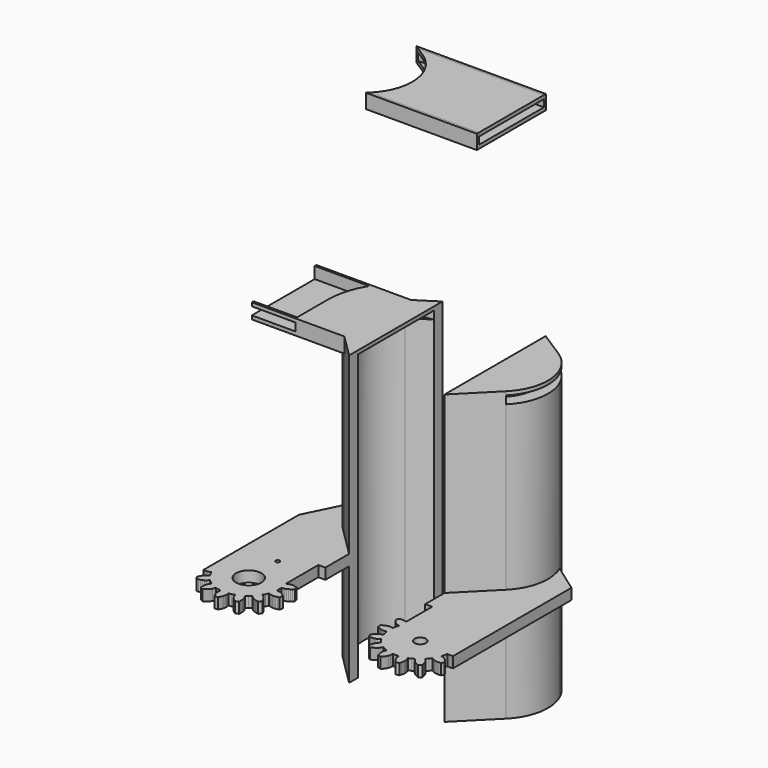
from build123d import *

# Parameters (mm, degrees)
F1_DEPTH  = 1.5
F0_R      = 1.6
F2_DEPTH  = 50
F3_DEPTH  = 30
F4_DEPTH  = 49
F5_DEPTH  = 46.8
F6_DEPTH  = 46.8
F7_DEPTH  = 45.8
F8_DEPTH  = 49
F9_DEPTH  = 45.8
F10_DEPTH = 1.5
F12_DEPTH = 4
F13_DEPTH = 3
F14_DEPTH = 1


# Not quite as in the source:
# - ends of sketch curves that miss each other by under 0.0002 mm in the source are joined
# - a feature names something its author has since deleted; it is built from what else it names


with BuildPart() as f1:
    # F0 (on Top) → F1 (new body, symmetric)
    with BuildSketch(Plane.XY):
        Polygon((-12.6828804, -37.9996929195), (-11.8884367355, -38.2222305677), (-11.8880267366, -38.2224279172), (-11.075543, -38.3664943195), (-11.1792258, -39.1773131195), (-11.1500412, -39.5862277195), (-11.049381, -40.0020257195), (-10.8967016, -40.4206431195), (-10.6978958, -40.8390065195), (-10.4565196, -41.2543727195), (-9.5434404, -41.2543727195), (-9.302115, -40.8390065195), (-9.1033092, -40.4206431195), (-8.950579, -40.0020257195), (-8.8499188, -39.5862277195), (-8.820785, -39.1773131195), (-8.9244678, -38.3664943195), (-8.1119840634, -38.2224279172), (-8.1115408, -38.2223493195), (-7.3171558, -37.9996929195), (-7.0589394, -38.7751549195), (-6.8550028, -39.1308311195), (-6.5838324, -39.4619201195), (-6.2647068, -39.7727145195), (-5.9041792, -40.0633667195), (-5.5066184, -40.3329369195), (-4.6838108, -39.9365445195), (-4.646549, -39.4578053195), (-4.6491144, -38.9947125195), (-4.693031, -38.5513555195), (-4.7828454, -38.1327635195), (-4.9339246, -37.7516365195), (-5.3789072, -37.0664715195), (-4.7096916266, -36.5840362135), (-4.709287, -36.5837445195), (-4.0899842, -36.0385589195), (-3.5209988, -36.6249941195), (-3.1831534, -36.8570993195), (-2.7948636, -37.0377695195), (-2.3725632, -37.1791713195), (-1.9218148, -37.2846829195), (-1.4464538, -37.3550663195), (-0.8770112, -36.6409453195), (-1.0512806, -36.1933973195), (-1.2544552, -35.7773199195), (-1.4865096, -35.3969041195), (-1.7489424, -35.0588555195), (-2.0504658, -34.7809287195), (-2.7488388, -34.3565455195), (-2.3551745142, -33.6315615111), (-2.3549356, -33.6311215195), (-2.0336002, -32.8714075195), (-1.2662154, -33.1527887195), (-0.86106, -33.2152727195), (-0.4331716, -33.2096847195), (0.0087884, -33.1539317195), (0.4607052, -33.0533223195), (0.9195562, -32.9104727195), (1.1227562, -32.0200757195), (0.7714742, -31.6924411195), (0.4079494, -31.4057259195), (0.033782, -31.1636639195), (-0.3494024, -30.9728083195), (-0.741426, -30.8533775195), (-1.5548356, -30.7739771195), (-1.5148031909, -29.9499745831), (-1.5147798, -29.9494931195), (-1.5548356, -29.1254663195), (-0.741426, -29.0460913195), (-0.3494024, -28.9266605195), (0.033782, -28.7358049195), (0.4079494, -28.4937683195), (0.7714742, -28.2070531195), (1.1227562, -27.8793931195), (0.9195562, -26.9889961195), (0.4607052, -26.8461465195), (0.0087884, -26.7455371195), (-0.4331716, -26.6898095195), (-0.86106, -26.6842215195), (-1.2662154, -26.7467055195), (-1.999996, -27.0157423195), (-1.999996, -15.8072914928), (-0.05, -15.8072914928), (-0.05, -8.999886363), (-7.8088611939, -1.2753778), (-20.002250767, -1.2753778), (-20.0087992, -33.1539317195), (-19.5667884, -33.2096847195), (-19.1389, -33.2152727195), (-18.7337954, -33.1527887195), (-17.9664106, -32.8714075195), (-17.6450069939, -33.6311141557), (-17.6448212, -33.6315533195), (-17.251172, -34.3565455195), (-17.9495196, -34.7809287195), (-18.2510684, -35.0588555195), (-18.5134504, -35.3969041195), (-18.745581, -35.7773199195), (-18.9487302, -36.1933973195), (-19.1229996, -36.6409453195), (-18.5535062, -37.3550663195), (-18.078196, -37.2846829195), (-17.6274476, -37.1791713195), (-17.2051218, -37.0377695195), (-16.8168066, -36.8570993195), (-16.479012, -36.6249941195), (-15.9100012, -36.0385589195), (-15.2906723648, -36.583686083), (-15.2903174, -36.5839985195), (-14.6211036, -37.0664715195), (-15.0660862, -37.7516365195), (-15.2171654, -38.1327635195), (-15.306929, -38.5513555195), (-15.3509218, -38.9947125195), (-15.3534618, -39.4578053195), (-15.3162, -39.9365445195), (-14.493367, -40.3329369195), (-14.0958062, -40.0633667195), (-13.735304, -39.7727145195), (-13.4161784, -39.4619201195), (-13.1449572, -39.1308311195), (-12.9410968, -38.7751549195), align=None)
        with BuildLine():
            ThreePointArc((-9.99998, -26.4247471195), (-7.5074285963, -27.4571957159), (-6.47498, -29.9497471195))
            ThreePointArc((-6.47498, -29.9497471195), (-12.4925314037, -32.4422985232), (-9.99998, -26.4247471195))
        make_face(mode=Mode.SUBTRACT)
        with BuildLine():
            ThreePointArc((-9.4549722, -19.9497471195), (-9.6146012888, -20.3351258307), (-9.99998, -20.4947549195))
            ThreePointArc((-9.99998, -20.4947549195), (-10.3853587112, -19.5643684084), (-9.4549722, -19.9497471195))
        make_face(mode=Mode.SUBTRACT)
        Polygon((-6.3914999282, -1.2753778), (-7.8088611939, -1.2753778), (-0.05, -8.999886363), (-0.05, -7.5888005143), align=None)
        Polygon((-8.4115295291, -0.6753778), (-7.8088611939, -1.2753778), (-6.3914999282, -1.2753778), (-6.9941682635, -0.6753778), align=None)
        with BuildLine():
            Line((-17.0059758203, 6.0612871152), (-17.0059758203, -0.6753778))
            Line((-17.0059758203, -0.6753778), (-8.4115295291, -0.6753778))
            Line((-8.4115295291, -0.6753778), (-6.9941682635, -0.6753778))
            Line((-6.9941682635, -0.6753778), (-8.8192027426, 1.1415762748))
            ThreePointArc((-8.8192027426, 1.1415762748), (-12.4595999549, 8.9958202972), (-10.1240431199, 17.331695494))
            Line((-10.1240431199, 17.331695494), (-12.1022985118, 15.9820039061))
            Line((-12.1022985118, 15.9820039061), (-17.0059758203, 6.0612871152))
        make_face()
        Polygon((-20.0019887813, 0), (-20.0021275162, -0.6753778), (-17.0059758203, -0.6753778), (-17.0059758203, 6.0612871152), align=None)
        Polygon((-20.0021275162, -0.6753778), (-20.002250767, -1.2753778), (-7.8088611939, -1.2753778), (-8.4115295291, -0.6753778), (-17.0059758203, -0.6753778), align=None)
    extrude(amount=F1_DEPTH, both=True)

    # F0 (on Top) → F2 (join)
    with BuildSketch(Plane.XY):
        with BuildLine():
            Line((-8.8192027426, 1.1415762748), (-6.9941682635, -0.6753778))
            Line((-6.9941682635, -0.6753778), (-0.05, -4.5405198881))
            Line((-0.05, -4.5405198881), (-7.28327834, 3.1477115777))
            ThreePointArc((-7.28327834, 3.1477115777), (-9.9219987158, 11.2465718924), (-5.3618740808, 18.4409896542))
            Line((-5.3618740808, 18.4409896542), (-0.05, 21.8151911543))
            Line((-0.05, 21.8151911543), (-6.7420944452, 20.5258809799))
            ThreePointArc((-6.7420944452, 20.5258809799), (-8.5829688524, 19.0874998536), (-10.1240431199, 17.331695494))
            ThreePointArc((-10.1240431199, 17.331695494), (-12.4595999549, 8.9958202972), (-8.8192027426, 1.1415762748))
        make_face()
        Polygon((-5.8053634872, 21.1258809799), (-6.7420944452, 20.5258809799), (-0.05, 21.8151911543), (-0.05, 22.999886363), (-0.05, 24.8123376548), align=None)
        Polygon((-6.9941682635, -0.6753778), (-6.3914999282, -1.2753778), (-0.05, -7.5888005143), (-0.05, -5.999886363), (-0.05, -4.5405198881), align=None)
        with BuildLine():
            Line((-7.28327834, 3.1477115777), (-0.05, -4.5405198881))
            Line((-0.05, -4.5405198881), (-0.05, 21.8151911543))
            Line((-0.05, 21.8151911543), (-5.3618740808, 18.4409896542))
            ThreePointArc((-5.3618740808, 18.4409896542), (-9.9219987158, 11.2465718924), (-7.28327834, 3.1477115777))
        make_face()
        with BuildLine():
            Line((-17.0059758203, 20.5258809799), (-17.0059758203, 6.0612871152))
            Line((-17.0059758203, 6.0612871152), (-12.1022985118, 15.9820039061))
            Line((-12.1022985118, 15.9820039061), (-10.1240431199, 17.331695494))
            ThreePointArc((-10.1240431199, 17.331695494), (-8.5829688524, 19.0874998536), (-6.7420944452, 20.5258809799))
            Line((-6.7420944452, 20.5258809799), (-17.0059758203, 20.5258809799))
        make_face()
        with BuildLine():
            Line((-19.9999346, 10), (-20.0019887813, 0))
            Line((-20.0019887813, 0), (-17.0059758203, 6.0612871152))
            Line((-17.0059758203, 6.0612871152), (-17.0059758203, 20.5258809799))
            ThreePointArc((-17.0059758203, 20.5258809799), (-19.2368888885, 15.4716989952), (-19.9999346, 10))
        make_face()
        Polygon((-20.0019887813, 0), (-20.0021275162, -0.6753778), (-17.0059758203, -0.6753778), (-17.0059758203, 6.0612871152), align=None)
        with BuildLine():
            Line((-17.0059758203, 6.0612871152), (-17.0059758203, -0.6753778))
            Line((-17.0059758203, -0.6753778), (-8.4115295291, -0.6753778))
            Line((-8.4115295291, -0.6753778), (-6.9941682635, -0.6753778))
            Line((-6.9941682635, -0.6753778), (-8.8192027426, 1.1415762748))
            ThreePointArc((-8.8192027426, 1.1415762748), (-12.4595999549, 8.9958202972), (-10.1240431199, 17.331695494))
            Line((-10.1240431199, 17.331695494), (-12.1022985118, 15.9820039061))
            Line((-12.1022985118, 15.9820039061), (-17.0059758203, 6.0612871152))
        make_face()
        with BuildLine():
            ThreePointArc((-16.6196316573, 21.1258809799), (-16.8154800574, 20.82760428), (-17.0059758203, 20.5258809799))
            Line((-17.0059758203, 20.5258809799), (-6.7420944452, 20.5258809799))
            Line((-6.7420944452, 20.5258809799), (-5.8053634872, 21.1258809799))
            Line((-5.8053634872, 21.1258809799), (-16.6196316573, 21.1258809799))
        make_face()
        Polygon((-8.4115295291, -0.6753778), (-7.8088611939, -1.2753778), (-6.3914999282, -1.2753778), (-6.9941682635, -0.6753778), align=None)
        Polygon((-20.0021275162, -0.6753778), (-20.002250767, -1.2753778), (-7.8088611939, -1.2753778), (-8.4115295291, -0.6753778), (-17.0059758203, -0.6753778), align=None)
        with BuildLine():
            Line((-27.5000003164, 20.5258809799), (-17.0059758203, 20.5258809799))
            ThreePointArc((-17.0059758203, 20.5258809799), (-16.8154800574, 20.82760428), (-16.6196316573, 21.1258809799))
            Line((-16.6196316573, 21.1258809799), (-27.5000003164, 21.1258809799))
            Line((-27.5000003164, 21.1258809799), (-32.0804677904, 21.1258809799))
            Line((-32.0804677904, 21.1258809799), (-32.0804677904, 20.5258809799))
            Line((-32.0804677904, 20.5258809799), (-27.5000003164, 20.5258809799))
        make_face()
        Polygon((-27.5000003164, -1.2753778), (-20.002250767, -1.2753778), (-20.0021275162, -0.6753778), (-27.5000003164, -0.6753778), (-32.0804677904, -0.6753778), (-32.0804677904, -1.2753778), align=None)
    extrude(amount=F2_DEPTH)

    # F0 (on Top) → F3 (join)
    with BuildSketch(Plane.XY):
        with BuildLine():
            Line((-8.8192027426, 1.1415762748), (-6.9941682635, -0.6753778))
            Line((-6.9941682635, -0.6753778), (-0.05, -4.5405198881))
            Line((-0.05, -4.5405198881), (-7.28327834, 3.1477115777))
            ThreePointArc((-7.28327834, 3.1477115777), (-9.9219987158, 11.2465718924), (-5.3618740808, 18.4409896542))
            Line((-5.3618740808, 18.4409896542), (-0.05, 21.8151911543))
            Line((-0.05, 21.8151911543), (-6.7420944452, 20.5258809799))
            ThreePointArc((-6.7420944452, 20.5258809799), (-8.5829688524, 19.0874998536), (-10.1240431199, 17.331695494))
            ThreePointArc((-10.1240431199, 17.331695494), (-12.4595999549, 8.9958202972), (-8.8192027426, 1.1415762748))
        make_face()
        Polygon((-6.9941682635, -0.6753778), (-6.3914999282, -1.2753778), (-0.05, -7.5888005143), (-0.05, -5.999886363), (-0.05, -4.5405198881), align=None)
        Polygon((-5.8053634872, 21.1258809799), (-6.7420944452, 20.5258809799), (-0.05, 21.8151911543), (-0.05, 22.999886363), (-0.05, 24.8123376548), align=None)
    extrude(amount=-F3_DEPTH)


with BuildPart() as f1b:
    # F0 (on Top) → F1, piece 2 (new body, symmetric)
    with BuildSketch(Plane.XY):
        with BuildLine():
            Line((45.5568809356, -32.5242657195), (45.7794119864, -31.729845607))
            Line((45.7794119864, -31.729845607), (45.7796203111, -31.7294128346))
            Line((45.7796203111, -31.7294128346), (45.9237077356, -30.9169283195))
            Line((45.9237077356, -30.9169283195), (46.7345011356, -31.0206111195))
            Line((46.7345011356, -31.0206111195), (47.1434157356, -30.9914519195))
            Line((47.1434157356, -30.9914519195), (47.5068643356, -30.9034663195))
            Line((47.5068643356, -30.9034663195), (47.5068643356, 10.1083564))
            Line((47.5068643356, 10.1083564), (39.8461772472, 15.5849402666))
            ThreePointArc((39.8461772472, 15.5849402666), (40.7766908436, 7.6257287323), (37.0316684565, 0.541259019))
            Line((37.0316684565, 0.541259019), (27.5569297356, -8.9911811067))
            Line((27.5569297356, -8.9911811067), (27.5569297356, -15.6989350928))
            Line((27.5569297356, -15.6989350928), (29.5069257356, -15.6989350928))
            Line((29.5069257356, -15.6989350928), (29.5069257356, -24.6967985195))
            Line((29.5069257356, -24.6967985195), (29.3238933356, -24.6242561195))
            Line((29.3238933356, -24.6242561195), (28.9053267356, -24.5344163195))
            Line((28.9053267356, -24.5344163195), (28.4619443356, -24.4904997195))
            Line((28.4619443356, -24.4904997195), (27.9988769356, -24.4879343195))
            Line((27.9988769356, -24.4879343195), (27.5201123356, -24.5252215195))
            Line((27.5201123356, -24.5252215195), (27.1237453356, -25.3480037195))
            Line((27.1237453356, -25.3480037195), (27.3933155356, -25.7455645195))
            Line((27.3933155356, -25.7455645195), (27.6839931356, -26.1060921195))
            Line((27.6839931356, -26.1060921195), (27.9947367356, -26.4252177195))
            Line((27.9947367356, -26.4252177195), (28.3259019356, -26.6964135195))
            Line((28.3259019356, -26.6964135195), (28.6815781356, -26.9003247195))
            Line((28.6815781356, -26.9003247195), (29.4569385356, -27.1585411195))
            Line((29.4569385356, -27.1585411195), (29.2345090358, -27.9529612023))
            Line((29.2345090358, -27.9529612023), (29.2343837356, -27.9534087195))
            Line((29.2343837356, -27.9534087195), (29.0901625356, -28.7658785195))
            Line((29.0901625356, -28.7658785195), (28.2793183356, -28.6621957195))
            Line((28.2793183356, -28.6621957195), (27.8704545356, -28.6913041195))
            Line((27.8704545356, -28.6913041195), (27.4546819356, -28.7919643195))
            Line((27.4546819356, -28.7919643195), (27.0360137356, -28.9447199195))
            Line((27.0360137356, -28.9447199195), (26.6177011356, -29.1435003195))
            Line((26.6177011356, -29.1435003195), (26.2023095356, -29.3848257195))
            Line((26.2023095356, -29.3848257195), (26.2023095356, -30.2979303195))
            Line((26.2023095356, -30.2979303195), (26.6177011356, -30.5392811195))
            Line((26.6177011356, -30.5392811195), (27.0360137356, -30.7380869195))
            Line((27.0360137356, -30.7380869195), (27.4546819356, -30.8907917195))
            Line((27.4546819356, -30.8907917195), (27.8704545356, -30.9914519195))
            Line((27.8704545356, -30.9914519195), (28.2793183356, -31.0206111195))
            Line((28.2793183356, -31.0206111195), (29.0901625356, -30.9169283195))
            Line((29.0901625356, -30.9169283195), (29.2343007326, -31.7294128446))
            Line((29.2343007326, -31.7294128446), (29.2343837356, -31.7298807195))
            Line((29.2343837356, -31.7298807195), (29.4569385356, -32.5242657195))
            Line((29.4569385356, -32.5242657195), (28.6815781356, -32.7824821195))
            Line((28.6815781356, -32.7824821195), (28.3259019356, -32.9863679195))
            Line((28.3259019356, -32.9863679195), (27.9947367356, -33.2575891195))
            Line((27.9947367356, -33.2575891195), (27.6839931356, -33.5766893195))
            Line((27.6839931356, -33.5766893195), (27.3933155356, -33.9371915195))
            Line((27.3933155356, -33.9371915195), (27.1237453356, -34.3347523195))
            Line((27.1237453356, -34.3347523195), (27.5201123356, -35.1575853195))
            Line((27.5201123356, -35.1575853195), (27.9988769356, -35.1948725195))
            Line((27.9988769356, -35.1948725195), (28.4619443356, -35.1923071195))
            Line((28.4619443356, -35.1923071195), (28.9053267356, -35.1483397195))
            Line((28.9053267356, -35.1483397195), (29.3238933356, -35.0585507195))
            Line((29.3238933356, -35.0585507195), (29.7050457356, -34.9074715195))
            Line((29.7050457356, -34.9074715195), (30.3902107356, -34.4624889195))
            Line((30.3902107356, -34.4624889195), (30.8726460484, -35.1317298871))
            Line((30.8726460484, -35.1317298871), (30.8729377356, -35.1321345195))
            Line((30.8729377356, -35.1321345195), (31.4180979356, -35.7513865195))
            Line((31.4180979356, -35.7513865195), (30.8316881356, -36.3203973195))
            Line((30.8316881356, -36.3203973195), (30.5995829356, -36.6582173195))
            Line((30.5995829356, -36.6582173195), (30.4189127356, -37.0465071195))
            Line((30.4189127356, -37.0465071195), (30.2775109356, -37.4688583195))
            Line((30.2775109356, -37.4688583195), (30.1719993356, -37.9196067195))
            Line((30.1719993356, -37.9196067195), (30.1016159356, -38.3949169195))
            Line((30.1016159356, -38.3949169195), (30.8157369356, -38.9643849195))
            Line((30.8157369356, -38.9643849195), (31.2632849356, -38.7901155195))
            Line((31.2632849356, -38.7901155195), (31.6793623356, -38.5869663195))
            Line((31.6793623356, -38.5869663195), (32.0597527356, -38.3548611195))
            Line((32.0597527356, -38.3548611195), (32.3978267356, -38.0924537195))
            Line((32.3978267356, -38.0924537195), (32.6757535356, -37.7909049195))
            Line((32.6757535356, -37.7909049195), (33.1001367356, -37.0925827195))
            Line((33.1001367356, -37.0925827195), (33.8251420267, -37.4861824058))
            Line((33.8251420267, -37.4861824058), (33.8255607356, -37.4864097195))
            Line((33.8255607356, -37.4864097195), (34.5852747356, -37.8077959195))
            Line((34.5852747356, -37.8077959195), (34.3038935356, -38.5752061195))
            Line((34.3038935356, -38.5752061195), (34.2414095356, -38.9803107195))
            Line((34.2414095356, -38.9803107195), (34.2469975356, -39.4081737195))
            Line((34.2469975356, -39.4081737195), (34.3027505356, -39.8501845195))
            Line((34.3027505356, -39.8501845195), (34.4033599356, -40.3021267195))
            Line((34.4033599356, -40.3021267195), (34.5461841356, -40.7609777195))
            Line((34.5461841356, -40.7609777195), (35.4366065356, -40.9641777195))
            Line((35.4366065356, -40.9641777195), (35.7642411356, -40.6128957195))
            Line((35.7642411356, -40.6128957195), (36.0509563356, -40.2493201195))
            Line((36.0509563356, -40.2493201195), (36.2929929356, -39.8751781195))
            Line((36.2929929356, -39.8751781195), (36.4838739356, -39.4919429195))
            Line((36.4838739356, -39.4919429195), (36.6033047356, -39.0999955195))
            Line((36.6033047356, -39.0999955195), (36.6826797356, -38.2865605195))
            Line((36.6826797356, -38.2865605195), (37.5067076121, -38.3265941598))
            Line((37.5067076121, -38.3265941598), (37.5071637356, -38.3266163195))
            Line((37.5071637356, -38.3266163195), (38.3311651356, -38.2865605195))
            Line((38.3311651356, -38.2865605195), (38.4105909356, -39.0999955195))
            Line((38.4105909356, -39.0999955195), (38.5299963356, -39.4919429195))
            Line((38.5299963356, -39.4919429195), (38.7208773356, -39.8751781195))
            Line((38.7208773356, -39.8751781195), (38.9629139356, -40.2493201195))
            Line((38.9629139356, -40.2493201195), (39.2496291356, -40.6128957195))
            Line((39.2496291356, -40.6128957195), (39.5772891356, -40.9641777195))
            Line((39.5772891356, -40.9641777195), (40.4676861356, -40.7609777195))
            Line((40.4676861356, -40.7609777195), (40.6105103356, -40.3021267195))
            Line((40.6105103356, -40.3021267195), (40.7111451356, -39.8501845195))
            Line((40.7111451356, -39.8501845195), (40.7668727356, -39.4081737195))
            Line((40.7668727356, -39.4081737195), (40.7724607356, -38.9803107195))
            Line((40.7724607356, -38.9803107195), (40.7099767356, -38.5752061195))
            Line((40.7099767356, -38.5752061195), (40.4285955356, -37.8077959195))
            Line((40.4285955356, -37.8077959195), (41.1883021717, -37.4863923134))
            Line((41.1883021717, -37.4863923134), (41.1887413356, -37.4862065195))
            Line((41.1887413356, -37.4862065195), (41.9137335356, -37.0925827195))
            Line((41.9137335356, -37.0925827195), (42.3381421356, -37.7909049195))
            Line((42.3381421356, -37.7909049195), (42.6160435356, -38.0924537195))
            Line((42.6160435356, -38.0924537195), (42.9541175356, -38.3548611195))
            Line((42.9541175356, -38.3548611195), (43.3345079356, -38.5869663195))
            Line((43.3345079356, -38.5869663195), (43.7505853356, -38.7901155195))
            Line((43.7505853356, -38.7901155195), (44.1981333356, -38.9643849195))
            Line((44.1981333356, -38.9643849195), (44.9122543356, -38.3949169195))
            Line((44.9122543356, -38.3949169195), (44.8418709356, -37.9196067195))
            Line((44.8418709356, -37.9196067195), (44.7363593356, -37.4688583195))
            Line((44.7363593356, -37.4688583195), (44.5949575356, -37.0465071195))
            Line((44.5949575356, -37.0465071195), (44.4142873356, -36.6582173195))
            Line((44.4142873356, -36.6582173195), (44.1821821356, -36.3203973195))
            Line((44.1821821356, -36.3203973195), (43.5957723356, -35.7513865195))
            Line((43.5957723356, -35.7513865195), (44.1408615089, -35.1320720054))
            Line((44.1408615089, -35.1320720054), (44.1411865356, -35.1317027195))
            Line((44.1411865356, -35.1317027195), (44.6236595356, -34.4624889195))
            Line((44.6236595356, -34.4624889195), (45.3088245356, -34.9074715195))
            Line((45.3088245356, -34.9074715195), (45.6899769356, -35.0585507195))
            Line((45.6899769356, -35.0585507195), (46.1085435356, -35.1483397195))
            Line((46.1085435356, -35.1483397195), (46.5519259356, -35.1923071195))
            Line((46.5519259356, -35.1923071195), (47.0149933356, -35.1948725195))
            Line((47.0149933356, -35.1948725195), (47.4937325356, -35.1575853195))
            Line((47.4937325356, -35.1575853195), (47.8901249356, -34.3347523195))
            Line((47.8901249356, -34.3347523195), (47.6205547356, -33.9371915195))
            Line((47.6205547356, -33.9371915195), (47.3299025356, -33.5766893195))
            Line((47.3299025356, -33.5766893195), (47.0191335356, -33.2575891195))
            Line((47.0191335356, -33.2575891195), (46.6880191356, -32.9863679195))
            Line((46.6880191356, -32.9863679195), (46.3323429356, -32.7824821195))
            Line((46.3323429356, -32.7824821195), (45.5568809356, -32.5242657195))
        make_face()
        with Locations((37.5069097356, -29.8413907195)):
            Circle(F0_R, mode=Mode.SUBTRACT)
    extrude(amount=F1_DEPTH, both=True)

    # F0 (on Top) → F2, piece 2 (join)
    with BuildSketch(Plane.XY):
        with BuildLine():
            Line((33.4049912244, 19.3934450196), (27.5569297356, 23.108242763))
            Line((27.5569297356, 23.108242763), (27.5569297356, 21.9235484419))
            Line((27.5569297356, 21.9235484419), (32.868804218, 18.5493466866))
            ThreePointArc((32.868804218, 18.5493466866), (37.4289291947, 11.3549283858), (34.7902086212, 3.2560674644))
            Line((34.7902086212, 3.2560674644), (32.236049682, 0.541259019))
            Line((32.236049682, 0.541259019), (33.609056732, 0.541259019))
            Line((33.609056732, 0.541259019), (35.5185359096, 2.5708391355))
            ThreePointArc((35.5185359096, 2.5708391355), (38.421128323, 11.4795854816), (33.4049912244, 19.3934450196))
        make_face()
        with BuildLine():
            ThreePointArc((37.0316684565, 0.541259019), (40.7766908436, 7.6257287323), (39.8461772472, 15.5849402666))
            ThreePointArc((39.8461772472, 15.5849402666), (37.7499815665, 18.9020978784), (34.788391552, 21.4763075705))
            Line((34.788391552, 21.4763075705), (32.2405845251, 23.108242763))
            Line((32.2405845251, 23.108242763), (27.5569297356, 23.108242763))
            Line((27.5569297356, 23.108242763), (33.4049912244, 19.3934450196))
            ThreePointArc((33.4049912244, 19.3934450196), (38.421128323, 11.4795854816), (35.5185359096, 2.5708391355))
            Line((35.5185359096, 2.5708391355), (33.609056732, 0.541259019))
            Line((33.609056732, 0.541259019), (37.0316684565, 0.541259019))
        make_face()
        with BuildLine():
            Line((32.868804218, 18.5493466866), (27.5569297356, 21.9235484419))
            Line((27.5569297356, 21.9235484419), (27.5569297356, -4.4321645815))
            Line((27.5569297356, -4.4321645815), (32.236049682, 0.541259019))
            Line((32.236049682, 0.541259019), (34.7902086212, 3.2560674644))
            ThreePointArc((34.7902086212, 3.2560674644), (37.4289291947, 11.3549283858), (32.868804218, 18.5493466866))
        make_face()
        Polygon((27.5569297356, -8.9911811067), (37.0316684565, 0.541259019), (33.609056732, 0.541259019), (27.5569297356, -5.891529963), align=None)
        Polygon((27.5569297356, -5.891529963), (33.609056732, 0.541259019), (32.236049682, 0.541259019), (27.5569297356, -4.4321645815), align=None)
        Polygon((32.2405845251, 23.108242763), (27.5569297356, 26.108242763), (27.5569297356, 23.108242763), align=None)
    extrude(amount=F2_DEPTH)

    # F0 (on Top) → F3, piece 2 (join)
    with BuildSketch(Plane.XY):
        with BuildLine():
            Line((33.4049912244, 19.3934450196), (27.5569297356, 23.108242763))
            Line((27.5569297356, 23.108242763), (27.5569297356, 21.9235484419))
            Line((27.5569297356, 21.9235484419), (32.868804218, 18.5493466866))
            ThreePointArc((32.868804218, 18.5493466866), (37.4289291947, 11.3549283858), (34.7902086212, 3.2560674644))
            Line((34.7902086212, 3.2560674644), (32.236049682, 0.541259019))
            Line((32.236049682, 0.541259019), (33.609056732, 0.541259019))
            Line((33.609056732, 0.541259019), (35.5185359096, 2.5708391355))
            ThreePointArc((35.5185359096, 2.5708391355), (38.421128323, 11.4795854816), (33.4049912244, 19.3934450196))
        make_face()
        with BuildLine():
            ThreePointArc((37.0316684565, 0.541259019), (40.7766908436, 7.6257287323), (39.8461772472, 15.5849402666))
            ThreePointArc((39.8461772472, 15.5849402666), (37.7499815665, 18.9020978784), (34.788391552, 21.4763075705))
            Line((34.788391552, 21.4763075705), (32.2405845251, 23.108242763))
            Line((32.2405845251, 23.108242763), (27.5569297356, 23.108242763))
            Line((27.5569297356, 23.108242763), (33.4049912244, 19.3934450196))
            ThreePointArc((33.4049912244, 19.3934450196), (38.421128323, 11.4795854816), (35.5185359096, 2.5708391355))
            Line((35.5185359096, 2.5708391355), (33.609056732, 0.541259019))
            Line((33.609056732, 0.541259019), (37.0316684565, 0.541259019))
        make_face()
        Polygon((27.5569297356, -8.9911811067), (37.0316684565, 0.541259019), (33.609056732, 0.541259019), (27.5569297356, -5.891529963), align=None)
        Polygon((27.5569297356, -5.891529963), (33.609056732, 0.541259019), (32.236049682, 0.541259019), (27.5569297356, -4.4321645815), align=None)
        Polygon((32.2405845251, 23.108242763), (27.5569297356, 26.108242763), (27.5569297356, 23.108242763), align=None)
    extrude(amount=-F3_DEPTH)


with BuildPart() as f4_tool:
    # F0 (on Top) → F4 (new body)
    with BuildSketch(Plane.XY):
        with BuildLine():
            Line((-8.8192027426, 1.1415762748), (-6.9941682635, -0.6753778))
            Line((-6.9941682635, -0.6753778), (-0.05, -4.5405198881))
            Line((-0.05, -4.5405198881), (-7.28327834, 3.1477115777))
            ThreePointArc((-7.28327834, 3.1477115777), (-9.9219987158, 11.2465718924), (-5.3618740808, 18.4409896542))
            Line((-5.3618740808, 18.4409896542), (-0.05, 21.8151911543))
            Line((-0.05, 21.8151911543), (-6.7420944452, 20.5258809799))
            ThreePointArc((-6.7420944452, 20.5258809799), (-8.5829688524, 19.0874998536), (-10.1240431199, 17.331695494))
            ThreePointArc((-10.1240431199, 17.331695494), (-12.4595999549, 8.9958202972), (-8.8192027426, 1.1415762748))
        make_face()
        with BuildLine():
            Line((-7.28327834, 3.1477115777), (-0.05, -4.5405198881))
            Line((-0.05, -4.5405198881), (-0.05, 21.8151911543))
            Line((-0.05, 21.8151911543), (-5.3618740808, 18.4409896542))
            ThreePointArc((-5.3618740808, 18.4409896542), (-9.9219987158, 11.2465718924), (-7.28327834, 3.1477115777))
        make_face()
        with BuildLine():
            Line((32.868804218, 18.5493466866), (27.5569297356, 21.9235484419))
            Line((27.5569297356, 21.9235484419), (27.5569297356, -4.4321645815))
            Line((27.5569297356, -4.4321645815), (32.236049682, 0.541259019))
            Line((32.236049682, 0.541259019), (34.7902086212, 3.2560674644))
            ThreePointArc((34.7902086212, 3.2560674644), (37.4289291947, 11.3549283858), (32.868804218, 18.5493466866))
        make_face()
        with BuildLine():
            Line((-19.9999346, 10), (-20.0019887813, 0))
            Line((-20.0019887813, 0), (-17.0059758203, 6.0612871152))
            Line((-17.0059758203, 6.0612871152), (-17.0059758203, 20.5258809799))
            ThreePointArc((-17.0059758203, 20.5258809799), (-19.2368888885, 15.4716989952), (-19.9999346, 10))
        make_face()
        Polygon((-20.0019887813, 0), (-20.0021275162, -0.6753778), (-17.0059758203, -0.6753778), (-17.0059758203, 6.0612871152), align=None)
        with BuildLine():
            Line((-17.0059758203, 6.0612871152), (-17.0059758203, -0.6753778))
            Line((-17.0059758203, -0.6753778), (-8.4115295291, -0.6753778))
            Line((-8.4115295291, -0.6753778), (-6.9941682635, -0.6753778))
            Line((-6.9941682635, -0.6753778), (-8.8192027426, 1.1415762748))
            ThreePointArc((-8.8192027426, 1.1415762748), (-12.4595999549, 8.9958202972), (-10.1240431199, 17.331695494))
            Line((-10.1240431199, 17.331695494), (-12.1022985118, 15.9820039061))
            Line((-12.1022985118, 15.9820039061), (-17.0059758203, 6.0612871152))
        make_face()
        with BuildLine():
            Line((-17.0059758203, 20.5258809799), (-17.0059758203, 6.0612871152))
            Line((-17.0059758203, 6.0612871152), (-12.1022985118, 15.9820039061))
            Line((-12.1022985118, 15.9820039061), (-10.1240431199, 17.331695494))
            ThreePointArc((-10.1240431199, 17.331695494), (-8.5829688524, 19.0874998536), (-6.7420944452, 20.5258809799))
            Line((-6.7420944452, 20.5258809799), (-17.0059758203, 20.5258809799))
        make_face()
        Polygon((-20.0021275162, -0.6753778), (-20.002250767, -1.2753778), (-7.8088611939, -1.2753778), (-8.4115295291, -0.6753778), (-17.0059758203, -0.6753778), align=None)
        Polygon((-8.4115295291, -0.6753778), (-7.8088611939, -1.2753778), (-6.3914999282, -1.2753778), (-6.9941682635, -0.6753778), align=None)
        with BuildLine():
            ThreePointArc((-16.6196316573, 21.1258809799), (-16.8154800574, 20.82760428), (-17.0059758203, 20.5258809799))
            Line((-17.0059758203, 20.5258809799), (-6.7420944452, 20.5258809799))
            Line((-6.7420944452, 20.5258809799), (-5.8053634872, 21.1258809799))
            Line((-5.8053634872, 21.1258809799), (-16.6196316573, 21.1258809799))
        make_face()
        with BuildLine():
            ThreePointArc((37.0316684565, 0.541259019), (40.7766908436, 7.6257287323), (39.8461772472, 15.5849402666))
            ThreePointArc((39.8461772472, 15.5849402666), (37.7499815665, 18.9020978784), (34.788391552, 21.4763075705))
            Line((34.788391552, 21.4763075705), (32.2405845251, 23.108242763))
            Line((32.2405845251, 23.108242763), (27.5569297356, 23.108242763))
            Line((27.5569297356, 23.108242763), (33.4049912244, 19.3934450196))
            ThreePointArc((33.4049912244, 19.3934450196), (38.421128323, 11.4795854816), (35.5185359096, 2.5708391355))
            Line((35.5185359096, 2.5708391355), (33.609056732, 0.541259019))
            Line((33.609056732, 0.541259019), (37.0316684565, 0.541259019))
        make_face()
        with BuildLine():
            Line((33.4049912244, 19.3934450196), (27.5569297356, 23.108242763))
            Line((27.5569297356, 23.108242763), (27.5569297356, 21.9235484419))
            Line((27.5569297356, 21.9235484419), (32.868804218, 18.5493466866))
            ThreePointArc((32.868804218, 18.5493466866), (37.4289291947, 11.3549283858), (34.7902086212, 3.2560674644))
            Line((34.7902086212, 3.2560674644), (32.236049682, 0.541259019))
            Line((32.236049682, 0.541259019), (33.609056732, 0.541259019))
            Line((33.609056732, 0.541259019), (35.5185359096, 2.5708391355))
            ThreePointArc((35.5185359096, 2.5708391355), (38.421128323, 11.4795854816), (33.4049912244, 19.3934450196))
        make_face()
        with BuildLine():
            Line((-27.5000003164, -0.6753778), (-20.0021275162, -0.6753778))
            Line((-20.0021275162, -0.6753778), (-20.0019887813, 0))
            Line((-20.0019887813, 0), (-19.9999346, 10))
            ThreePointArc((-19.9999346, 10), (-19.2368888885, 15.4716989952), (-17.0059758203, 20.5258809799))
            Line((-17.0059758203, 20.5258809799), (-27.5000003164, 20.5258809799))
            Line((-27.5000003164, 20.5258809799), (-32.0804677904, 20.5258809799))
            Line((-32.0804677904, 20.5258809799), (-32.0804677904, -0.6753778))
            Line((-32.0804677904, -0.6753778), (-27.5000003164, -0.6753778))
        make_face()
        Polygon((-27.5000003164, -1.2753778), (-20.002250767, -1.2753778), (-20.0021275162, -0.6753778), (-27.5000003164, -0.6753778), (-32.0804677904, -0.6753778), (-32.0804677904, -1.2753778), align=None)
    extrude(amount=F4_DEPTH)


with BuildPart() as f1_1:
    add(f1.part)

    # F4: cut by f4_tool
    add(f4_tool.part, mode=Mode.SUBTRACT)

    # F0 (on Top) → F5, piece 2 (join)
    with BuildSketch(Plane.XY):
        with BuildLine():
            Line((-8.8192027426, 1.1415762748), (-6.9941682635, -0.6753778))
            Line((-6.9941682635, -0.6753778), (-0.05, -4.5405198881))
            Line((-0.05, -4.5405198881), (-7.28327834, 3.1477115777))
            ThreePointArc((-7.28327834, 3.1477115777), (-9.9219987158, 11.2465718924), (-5.3618740808, 18.4409896542))
            Line((-5.3618740808, 18.4409896542), (-0.05, 21.8151911543))
            Line((-0.05, 21.8151911543), (-6.7420944452, 20.5258809799))
            ThreePointArc((-6.7420944452, 20.5258809799), (-8.5829688524, 19.0874998536), (-10.1240431199, 17.331695494))
            ThreePointArc((-10.1240431199, 17.331695494), (-12.4595999549, 8.9958202972), (-8.8192027426, 1.1415762748))
        make_face()
        Polygon((-27.5000003164, -1.2753778), (-20.002250767, -1.2753778), (-20.0021275162, -0.6753778), (-27.5000003164, -0.6753778), (-32.0804677904, -0.6753778), (-32.0804677904, -1.2753778), align=None)
    extrude(amount=F5_DEPTH)

    # F0 (on Top) → F6 (join)
    with BuildSketch(Plane.XY):
        Polygon((-20.0019887813, 0), (-20.0021275162, -0.6753778), (-17.0059758203, -0.6753778), (-17.0059758203, 6.0612871152), align=None)
        with BuildLine():
            Line((-19.9999346, 10), (-20.0019887813, 0))
            Line((-20.0019887813, 0), (-17.0059758203, 6.0612871152))
            Line((-17.0059758203, 6.0612871152), (-17.0059758203, 20.5258809799))
            ThreePointArc((-17.0059758203, 20.5258809799), (-19.2368888885, 15.4716989952), (-19.9999346, 10))
        make_face()
        with BuildLine():
            Line((-17.0059758203, 20.5258809799), (-17.0059758203, 6.0612871152))
            Line((-17.0059758203, 6.0612871152), (-12.1022985118, 15.9820039061))
            Line((-12.1022985118, 15.9820039061), (-10.1240431199, 17.331695494))
            ThreePointArc((-10.1240431199, 17.331695494), (-8.5829688524, 19.0874998536), (-6.7420944452, 20.5258809799))
            Line((-6.7420944452, 20.5258809799), (-17.0059758203, 20.5258809799))
        make_face()
        with BuildLine():
            Line((-17.0059758203, 6.0612871152), (-17.0059758203, -0.6753778))
            Line((-17.0059758203, -0.6753778), (-8.4115295291, -0.6753778))
            Line((-8.4115295291, -0.6753778), (-6.9941682635, -0.6753778))
            Line((-6.9941682635, -0.6753778), (-8.8192027426, 1.1415762748))
            ThreePointArc((-8.8192027426, 1.1415762748), (-12.4595999549, 8.9958202972), (-10.1240431199, 17.331695494))
            Line((-10.1240431199, 17.331695494), (-12.1022985118, 15.9820039061))
            Line((-12.1022985118, 15.9820039061), (-17.0059758203, 6.0612871152))
        make_face()
        with BuildLine():
            Line((-27.5000003164, -0.6753778), (-20.0021275162, -0.6753778))
            Line((-20.0021275162, -0.6753778), (-20.0019887813, 0))
            Line((-20.0019887813, 0), (-19.9999346, 10))
            ThreePointArc((-19.9999346, 10), (-19.2368888885, 15.4716989952), (-17.0059758203, 20.5258809799))
            Line((-17.0059758203, 20.5258809799), (-27.5000003164, 20.5258809799))
            Line((-27.5000003164, 20.5258809799), (-32.0804677904, 20.5258809799))
            Line((-32.0804677904, 20.5258809799), (-32.0804677904, -0.6753778))
            Line((-32.0804677904, -0.6753778), (-27.5000003164, -0.6753778))
        make_face()
        Polygon((-27.5000003164, -1.2753778), (-20.002250767, -1.2753778), (-20.0021275162, -0.6753778), (-27.5000003164, -0.6753778), (-32.0804677904, -0.6753778), (-32.0804677904, -1.2753778), align=None)
        Polygon((-20.0021275162, -0.6753778), (-20.002250767, -1.2753778), (-7.8088611939, -1.2753778), (-8.4115295291, -0.6753778), (-17.0059758203, -0.6753778), align=None)
    extrude(amount=F6_DEPTH)

    # F0 (on Top) → F7 (cut)
    with BuildSketch(Plane.XY):
        Polygon((-20.0019887813, 0), (-20.0021275162, -0.6753778), (-17.0059758203, -0.6753778), (-17.0059758203, 6.0612871152), align=None)
        with BuildLine():
            Line((-17.0059758203, 6.0612871152), (-17.0059758203, -0.6753778))
            Line((-17.0059758203, -0.6753778), (-8.4115295291, -0.6753778))
            Line((-8.4115295291, -0.6753778), (-6.9941682635, -0.6753778))
            Line((-6.9941682635, -0.6753778), (-8.8192027426, 1.1415762748))
            ThreePointArc((-8.8192027426, 1.1415762748), (-12.4595999549, 8.9958202972), (-10.1240431199, 17.331695494))
            Line((-10.1240431199, 17.331695494), (-12.1022985118, 15.9820039061))
            Line((-12.1022985118, 15.9820039061), (-17.0059758203, 6.0612871152))
        make_face()
        with BuildLine():
            Line((-19.9999346, 10), (-20.0019887813, 0))
            Line((-20.0019887813, 0), (-17.0059758203, 6.0612871152))
            Line((-17.0059758203, 6.0612871152), (-17.0059758203, 20.5258809799))
            ThreePointArc((-17.0059758203, 20.5258809799), (-19.2368888885, 15.4716989952), (-19.9999346, 10))
        make_face()
        with BuildLine():
            Line((-17.0059758203, 20.5258809799), (-17.0059758203, 6.0612871152))
            Line((-17.0059758203, 6.0612871152), (-12.1022985118, 15.9820039061))
            Line((-12.1022985118, 15.9820039061), (-10.1240431199, 17.331695494))
            ThreePointArc((-10.1240431199, 17.331695494), (-8.5829688524, 19.0874998536), (-6.7420944452, 20.5258809799))
            Line((-6.7420944452, 20.5258809799), (-17.0059758203, 20.5258809799))
        make_face()
        with BuildLine():
            Line((-27.5000003164, -0.6753778), (-20.0021275162, -0.6753778))
            Line((-20.0021275162, -0.6753778), (-20.0019887813, 0))
            Line((-20.0019887813, 0), (-19.9999346, 10))
            ThreePointArc((-19.9999346, 10), (-19.2368888885, 15.4716989952), (-17.0059758203, 20.5258809799))
            Line((-17.0059758203, 20.5258809799), (-27.5000003164, 20.5258809799))
            Line((-27.5000003164, 20.5258809799), (-32.0804677904, 20.5258809799))
            Line((-32.0804677904, 20.5258809799), (-32.0804677904, -0.6753778))
            Line((-32.0804677904, -0.6753778), (-27.5000003164, -0.6753778))
        make_face()
        Polygon((-27.5000003164, -1.2753778), (-20.002250767, -1.2753778), (-20.0021275162, -0.6753778), (-27.5000003164, -0.6753778), (-32.0804677904, -0.6753778), (-32.0804677904, -1.2753778), align=None)
        with BuildLine():
            Line((-27.5000003164, 20.5258809799), (-17.0059758203, 20.5258809799))
            ThreePointArc((-17.0059758203, 20.5258809799), (-16.8154800574, 20.82760428), (-16.6196316573, 21.1258809799))
            Line((-16.6196316573, 21.1258809799), (-27.5000003164, 21.1258809799))
            Line((-27.5000003164, 21.1258809799), (-32.0804677904, 21.1258809799))
            Line((-32.0804677904, 21.1258809799), (-32.0804677904, 20.5258809799))
            Line((-32.0804677904, 20.5258809799), (-27.5000003164, 20.5258809799))
        make_face()
    extrude(amount=F7_DEPTH, mode=Mode.SUBTRACT)

    # F0 (on Top) → F8 (join)
    with BuildSketch(Plane.XY):
        Polygon((-8.4115295291, -0.6753778), (-7.8088611939, -1.2753778), (-6.3914999282, -1.2753778), (-6.9941682635, -0.6753778), align=None)
        Polygon((-20.0021275162, -0.6753778), (-20.002250767, -1.2753778), (-7.8088611939, -1.2753778), (-8.4115295291, -0.6753778), (-17.0059758203, -0.6753778), align=None)
        with BuildLine():
            ThreePointArc((-16.6196316573, 21.1258809799), (-16.8154800574, 20.82760428), (-17.0059758203, 20.5258809799))
            Line((-17.0059758203, 20.5258809799), (-6.7420944452, 20.5258809799))
            Line((-6.7420944452, 20.5258809799), (-5.8053634872, 21.1258809799))
            Line((-5.8053634872, 21.1258809799), (-16.6196316573, 21.1258809799))
        make_face()
    extrude(amount=F8_DEPTH)

    # F0 (on Top) → F9 (cut)
    with BuildSketch(Plane.XY):
        Polygon((-8.4115295291, -0.6753778), (-7.8088611939, -1.2753778), (-6.3914999282, -1.2753778), (-6.9941682635, -0.6753778), align=None)
        Polygon((-20.0021275162, -0.6753778), (-20.002250767, -1.2753778), (-7.8088611939, -1.2753778), (-8.4115295291, -0.6753778), (-17.0059758203, -0.6753778), align=None)
        with BuildLine():
            ThreePointArc((-16.6196316573, 21.1258809799), (-16.8154800574, 20.82760428), (-17.0059758203, 20.5258809799))
            Line((-17.0059758203, 20.5258809799), (-6.7420944452, 20.5258809799))
            Line((-6.7420944452, 20.5258809799), (-5.8053634872, 21.1258809799))
            Line((-5.8053634872, 21.1258809799), (-16.6196316573, 21.1258809799))
        make_face()
    extrude(amount=F9_DEPTH, mode=Mode.SUBTRACT)

    # F0 (on Top) → F10 (join)
    with BuildSketch(Plane.XY):
        Polygon((-20.0019887813, 0), (-20.0021275162, -0.6753778), (-17.0059758203, -0.6753778), (-17.0059758203, 6.0612871152), align=None)
        with BuildLine():
            Line((-17.0059758203, 6.0612871152), (-17.0059758203, -0.6753778))
            Line((-17.0059758203, -0.6753778), (-8.4115295291, -0.6753778))
            Line((-8.4115295291, -0.6753778), (-6.9941682635, -0.6753778))
            Line((-6.9941682635, -0.6753778), (-8.8192027426, 1.1415762748))
            ThreePointArc((-8.8192027426, 1.1415762748), (-12.4595999549, 8.9958202972), (-10.1240431199, 17.331695494))
            Line((-10.1240431199, 17.331695494), (-12.1022985118, 15.9820039061))
            Line((-12.1022985118, 15.9820039061), (-17.0059758203, 6.0612871152))
        make_face()
        Polygon((-20.0021275162, -0.6753778), (-20.002250767, -1.2753778), (-7.8088611939, -1.2753778), (-8.4115295291, -0.6753778), (-17.0059758203, -0.6753778), align=None)
        Polygon((-8.4115295291, -0.6753778), (-7.8088611939, -1.2753778), (-6.3914999282, -1.2753778), (-6.9941682635, -0.6753778), align=None)
    extrude(amount=F10_DEPTH)


with BuildPart() as f1b_1:
    add(f1b.part)

    # F4: cut by f4_tool
    add(f4_tool.part, mode=Mode.SUBTRACT)

    # F0 (on Top) → F5 (join)
    with BuildSketch(Plane.XY):
        with BuildLine():
            ThreePointArc((37.0316684565, 0.541259019), (40.7766908436, 7.6257287323), (39.8461772472, 15.5849402666))
            ThreePointArc((39.8461772472, 15.5849402666), (37.7499815665, 18.9020978784), (34.788391552, 21.4763075705))
            Line((34.788391552, 21.4763075705), (32.2405845251, 23.108242763))
            Line((32.2405845251, 23.108242763), (27.5569297356, 23.108242763))
            Line((27.5569297356, 23.108242763), (33.4049912244, 19.3934450196))
            ThreePointArc((33.4049912244, 19.3934450196), (38.421128323, 11.4795854816), (35.5185359096, 2.5708391355))
            Line((35.5185359096, 2.5708391355), (33.609056732, 0.541259019))
            Line((33.609056732, 0.541259019), (37.0316684565, 0.541259019))
        make_face()
        with BuildLine():
            Line((33.4049912244, 19.3934450196), (27.5569297356, 23.108242763))
            Line((27.5569297356, 23.108242763), (27.5569297356, 21.9235484419))
            Line((27.5569297356, 21.9235484419), (32.868804218, 18.5493466866))
            ThreePointArc((32.868804218, 18.5493466866), (37.4289291947, 11.3549283858), (34.7902086212, 3.2560674644))
            Line((34.7902086212, 3.2560674644), (32.236049682, 0.541259019))
            Line((32.236049682, 0.541259019), (33.609056732, 0.541259019))
            Line((33.609056732, 0.541259019), (35.5185359096, 2.5708391355))
            ThreePointArc((35.5185359096, 2.5708391355), (38.421128323, 11.4795854816), (33.4049912244, 19.3934450196))
        make_face()
    extrude(amount=F5_DEPTH)


with BuildPart() as f12:
    # F11 (on face) → F12 (new body)
    with BuildSketch(Plane.XY.offset(50)):
        Polygon((-63.4200498444, 91.6449610588), (-73.5252730212, 91.6449610588), (-74.2159536496, 90.9500741675), (-63.4200498444, 90.9500741675), (-43.4200498444, 90.9500741675), (-43.4200498444, 91.6449610588), align=None)
        Polygon((-79.3612307015, 114.8812130107), (-78.3230413675, 114.2162263407), (-63.4200498444, 114.2162263407), (-43.4200498444, 114.2162263407), (-43.4200498444, 114.8812130107), (-63.4200498444, 114.8812130107), align=None)
        with BuildLine():
            Line((-63.4200498444, 114.2162263407), (-78.3230413675, 114.2162263407))
            Line((-78.3230413675, 114.2162263407), (-75.7685499257, 112.5800096104))
            ThreePointArc((-75.7685499257, 112.5800096104), (-69.626854193, 102.6504052027), (-73.5252730212, 91.6449610588))
            Line((-73.5252730212, 91.6449610588), (-63.4200498444, 91.6449610588))
            Line((-63.4200498444, 91.6449610588), (-43.4200498444, 91.6449610588))
            Line((-43.4200498444, 91.6449610588), (-43.4200498444, 114.2162263407))
            Line((-43.4200498444, 114.2162263407), (-63.4200498444, 114.2162263407))
        make_face()
    extrude(amount=-F12_DEPTH)

    # F11 (on face) → F13 (cut)
    with BuildSketch(Plane.XY.offset(50)):
        with BuildLine():
            Line((-63.4200498444, 114.2162263407), (-78.3230413675, 114.2162263407))
            Line((-78.3230413675, 114.2162263407), (-75.7685499257, 112.5800096104))
            ThreePointArc((-75.7685499257, 112.5800096104), (-69.626854193, 102.6504052027), (-73.5252730212, 91.6449610588))
            Line((-73.5252730212, 91.6449610588), (-63.4200498444, 91.6449610588))
            Line((-63.4200498444, 91.6449610588), (-43.4200498444, 91.6449610588))
            Line((-43.4200498444, 91.6449610588), (-43.4200498444, 114.2162263407))
            Line((-43.4200498444, 114.2162263407), (-63.4200498444, 114.2162263407))
        make_face()
    extrude(amount=-F13_DEPTH, mode=Mode.SUBTRACT)


with BuildPart() as f14:
    # F11 (on face) → F14 (new body)
    with BuildSketch(Plane.XY.offset(50)):
        with BuildLine():
            Line((-63.4200498444, 114.2162263407), (-78.3230413675, 114.2162263407))
            Line((-78.3230413675, 114.2162263407), (-75.7685499257, 112.5800096104))
            ThreePointArc((-75.7685499257, 112.5800096104), (-69.626854193, 102.6504052027), (-73.5252730212, 91.6449610588))
            Line((-73.5252730212, 91.6449610588), (-63.4200498444, 91.6449610588))
            Line((-63.4200498444, 91.6449610588), (-43.4200498444, 91.6449610588))
            Line((-43.4200498444, 91.6449610588), (-43.4200498444, 114.2162263407))
            Line((-43.4200498444, 114.2162263407), (-63.4200498444, 114.2162263407))
        make_face()
    extrude(amount=-F14_DEPTH)


solid = Compound([f1_1.part, f1b_1.part, f12.part, f14.part])
